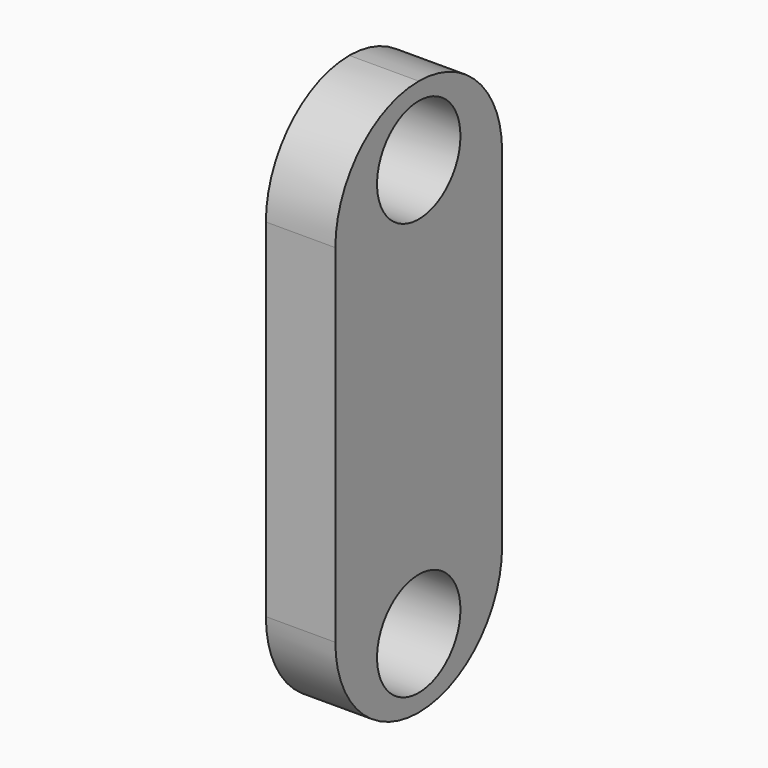
from build123d import *

# Parameters (mm, degrees)
F0_W     = 19.05
F0_H     = 50.8
F0_R     = 4.7625
F1_DEPTH = 6.35
F2_R     = 9.52499


# Not quite as in the source:
# - a fillet or chamfer is up to 0.001 mm smaller than in the source, because OpenCascade refuses the exact size


with BuildPart() as f1:
    # F0 (on Right) → F1 (new body)
    with BuildSketch(Plane.YZ):
        Rectangle(F0_W, F0_H)
        with Locations((0, -19.05)):
            Circle(F0_R, mode=Mode.SUBTRACT)
        with Locations((0, 19.05)):
            Circle(F0_R, mode=Mode.SUBTRACT)
    extrude(amount=F1_DEPTH)

    # F2 (radius 9.525 in the source; OpenCascade refuses exactly that, so slightly less here)
    f2_edges = [f1.edges().sort_by_distance(p)[0] for p in [
        (3.175, 9.525, 25.4),
        (3.175, -9.525, 25.4),
        (3.175, 9.525, -25.4),
        (3.175, -9.525, -25.4),
    ]]
    fillet(f2_edges, radius=F2_R)


solid = f1.part
